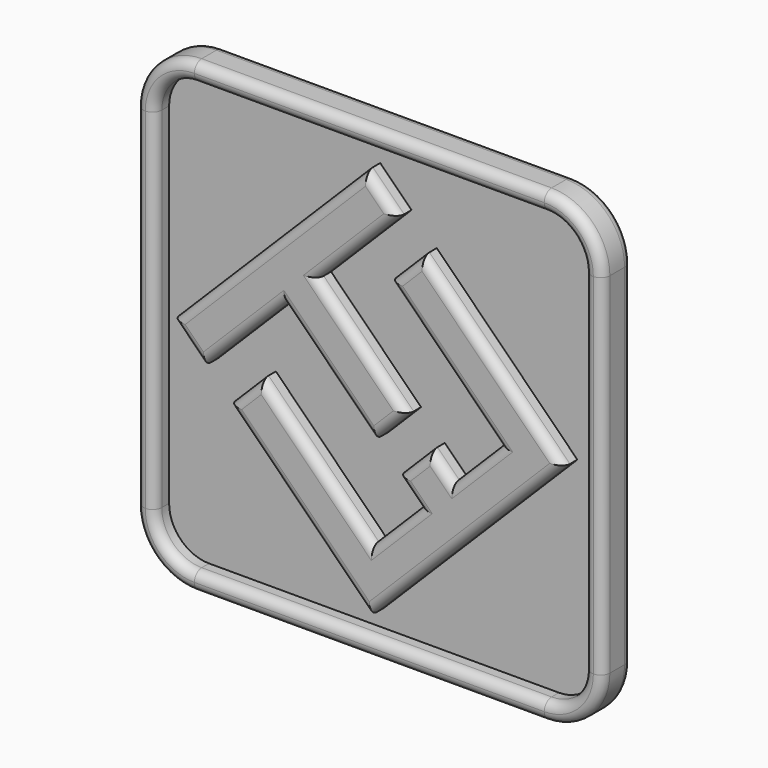
from build123d import *

# Parameters (mm, degrees)
F1_DEPTH = 1.5
F2_DEPTH = 3
F4_DEPTH = 3
F5_R     = 0.74999
F6_R     = 0.75


# Not quite as in the source:
# - a fillet or chamfer is up to 0.001 mm smaller than in the source, because OpenCascade refuses the exact size


with BuildPart() as f1:
    # F0 (on Front) → F1 (new body)
    with BuildSketch(Plane.XZ):
        with BuildLine():
            ThreePointArc((-19.05, -14.2875), (-17.6550960454, -17.6550960454), (-14.2875, -19.05))
            Line((-14.2875, -19.05), (14.2875, -19.05))
            ThreePointArc((14.2875, -19.05), (17.6550960454, -17.6550960454), (19.05, -14.2875))
            Line((19.05, -14.2875), (19.05, 14.2875))
            ThreePointArc((19.05, 14.2875), (17.6550960454, 17.6550960454), (14.2875, 19.05))
            Line((14.2875, 19.05), (-14.2875, 19.05))
            ThreePointArc((-14.2875, 19.05), (-17.6550960454, 17.6550960454), (-19.05, 14.2875))
            Line((-19.05, 14.2875), (-19.05, -14.2875))
        make_face()
        Polygon((15.791487975, -0.306085875), (0, -16.09757385), (-11.48107305, -4.616510325), (-8.829722625, -1.9651599), (0.16503015, -10.95990315), (4.083738975, -7.0411848), (2.315441775, -5.2728876), (4.9667922, -2.621537175), (6.735098925, -4.389834375), (10.65380775, -0.471116025), (1.6590645, 8.523627225), (4.310414925, 11.17497765), align=None, mode=Mode.SUBTRACT)
        Polygon((-6.975852825, 4.018416525), (-13.5459216, -2.55165225), (-16.09757385, 0), (-0.306085875, 15.791487975), (2.245566375, 13.239835725), (-4.3245024, 6.66976695), (3.025206675, -0.679942125), (0.37385625, -3.331302075), align=None, mode=Mode.SUBTRACT)
    extrude(amount=F1_DEPTH)

    # F0 (on Front) → F2 (join)
    with BuildSketch(Plane.XZ):
        Polygon((-16.09757385, 0), (-13.5459216, -2.55165225), (-6.975852825, 4.018416525), (0.37385625, -3.331302075), (3.025206675, -0.679942125), (-4.3245024, 6.66976695), (2.245566375, 13.239835725), (-0.306085875, 15.791487975), align=None)
        Polygon((-11.48107305, -4.616510325), (0, -16.09757385), (15.791487975, -0.306085875), (4.310414925, 11.17497765), (1.6590645, 8.523627225), (10.65380775, -0.471116025), (6.735098925, -4.389834375), (4.9667922, -2.621537175), (2.315441775, -5.2728876), (4.083738975, -7.0411848), (0.16503015, -10.95990315), (-8.829722625, -1.9651599), align=None)
    extrude(amount=F2_DEPTH)

    # F3 (on face) → F4 (join)
    with BuildSketch(Plane.XZ):
        with BuildLine():
            ThreePointArc((-14.2875, 19.05), (-17.6550960454, 17.6550960454), (-19.05, 14.2875))
            Line((-19.05, 14.2875), (-19.05, -14.2875))
            ThreePointArc((-19.05, -14.2875), (-17.6550960454, -17.6550960454), (-14.2875, -19.05))
            Line((-14.2875, -19.05), (14.2875, -19.05))
            ThreePointArc((14.2875, -19.05), (17.6550960454, -17.6550960454), (19.05, -14.2875))
            Line((19.05, -14.2875), (19.05, 14.2875))
            ThreePointArc((19.05, 14.2875), (17.6550960454, 17.6550960454), (14.2875, 19.05))
            Line((14.2875, 19.05), (-14.2875, 19.05))
        make_face()
        with BuildLine():
            ThreePointArc((-17.55, 14.2875), (-16.5944358736, 16.5944358736), (-14.2875, 17.55))
            Line((-14.2875, 17.55), (14.2875, 17.55))
            ThreePointArc((14.2875, 17.55), (16.5944358736, 16.5944358736), (17.55, 14.2875))
            Line((17.55, 14.2875), (17.55, -14.2875))
            ThreePointArc((17.55, -14.2875), (16.5944358736, -16.5944358736), (14.2875, -17.55))
            Line((14.2875, -17.55), (-14.2875, -17.55))
            ThreePointArc((-14.2875, -17.55), (-16.5944358736, -16.5944358736), (-17.55, -14.2875))
            Line((-17.55, -14.2875), (-17.55, 14.2875))
        make_face(mode=Mode.SUBTRACT)
    extrude(amount=F4_DEPTH)

    # F5 (radius 0.75 in the source; OpenCascade refuses exactly that, so slightly less here)
    f5_edges = [f1.edges().sort_by_distance(p)[0] for p in [
        (-4.332346, -3, -6.462532),
        (-10.155398, -3, -3.290835),
        (-5.740537, -3, -10.357042),
        (7.895744, -3, -8.20183),
        (10.050951, -3, 5.434446),
        (2.98474, -3, 9.849302),
        (6.156436, -3, 4.026256),
        (8.694453, -3, -2.430475),
        (5.850946, -3, -3.505686),
        (3.641117, -3, -3.947212),
        (3.19959, -3, -6.157036),
        (2.124385, -3, -9.000544),
        (-8.20183, -3, 7.895744),
        (-14.821748, -3, -1.275826),
        (-10.260887, -3, 0.733382),
        (-3.300998, -3, 0.343557),
        (1.699531, -3, -2.005622),
        (-0.649648, -3, 2.994912),
        (-1.039468, -3, 9.954801),
        (0.96974, -3, 14.515662),
        (-17.655096, -3, 17.655096),
        (-19.05, -3, 0),
        (-17.655096, -3, -17.655096),
        (0, -3, -19.05),
        (17.655096, -3, -17.655096),
        (19.05, -3, 0),
        (17.655096, -3, 17.655096),
        (0, -3, 19.05),
        (-16.594436, -3, 16.594436),
        (0, -3, 17.55),
        (16.594436, -3, 16.594436),
        (17.55, -3, 0),
        (16.594436, -3, -16.594436),
        (0, -3, -17.55),
        (-16.594436, -3, -16.594436),
        (-17.55, -3, 0),
    ]]
    fillet(f5_edges, radius=F5_R)

    # F6
    f6_edges = [f1.edges().sort_by_distance(p)[0] for p in [
        (-17.655096, 0, -17.655096),
        (0, 0, -19.05),
        (17.655096, 0, -17.655096),
        (19.05, 0, 0),
        (17.655096, 0, 17.655096),
        (0, 0, 19.05),
        (-17.655096, 0, 17.655096),
        (-19.05, 0, 0),
    ]]
    fillet(f6_edges, radius=F6_R)


solid = f1.part
